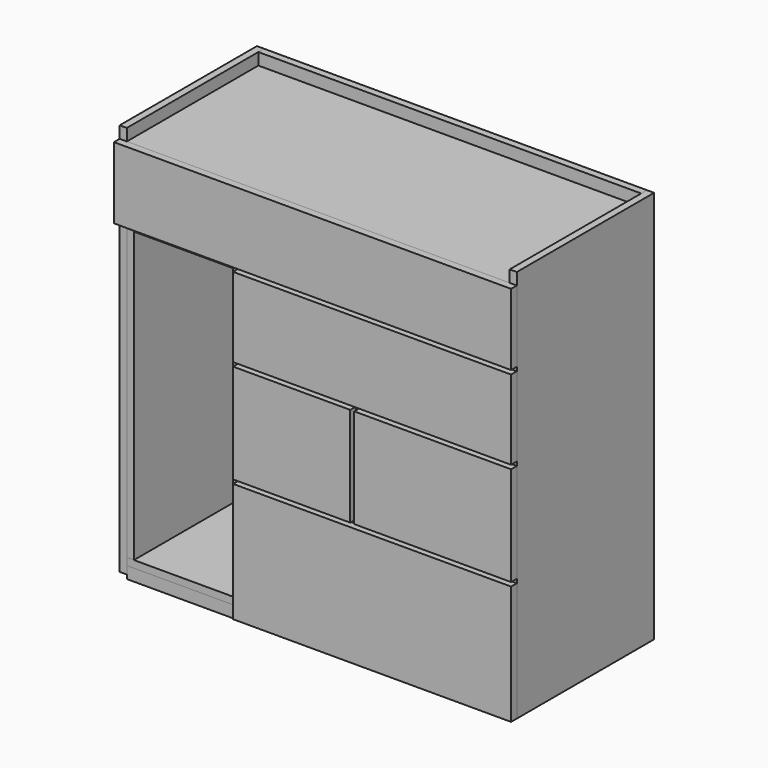
from build123d import *

# Parameters (mm, degrees)
F0_W          = 18
F0_H          = 414
F0_H_2        = 18
F1_DEPTH      = 990
F0_W_2        = 964
F2_DEPTH      = 990
F3_DEPTH      = 20
F3_DEPTH_BACK = 10
F4_W          = 982
F4_H          = 180
F4_W_2        = 18
F5_DEPTH      = 18
F4_W_3        = 700
F4_H_2        = 200
F4_W_4        = 395
F4_H_3        = 250
F4_H_4        = 300
F4_W_5        = 295
F6_W          = 964
F6_H          = 18
F7_DEPTH      = 414
F6_H_2        = 4
F6_W_2        = 18
F6_W_3        = 250
F6_H_3        = 192
F6_H_4        = 258
F6_H_5        = 242
F8_DEPTH      = 414
F9_R          = 10
F10_DEPTH     = 250
F11_W         = 250
F11_H         = 728
F12_DEPTH     = 12


# Not quite as in the source:
# - a feature names something its author has since deleted; it is built from what else it names


with BuildPart() as f1:
    # F0 (on Top) → F1 (new body)
    with BuildSketch(Plane.XY):
        with Locations((9, 207)):
            Rectangle(F0_W, F0_H)
        with Locations((9, 423)):
            Rectangle(F0_W, F0_H_2)
    extrude(amount=F1_DEPTH)


with BuildPart() as f1b:
    # F0 (on Top) → F1, piece 2 (new body)
    with BuildSketch(Plane.XY):
        with Locations((991, 423)):
            Rectangle(F0_W, F0_H_2)
        with Locations((991, 207)):
            Rectangle(F0_W, F0_H)
    extrude(amount=F1_DEPTH)


with BuildPart() as f2:
    # F0 (on Top) → F2 (new body, through all)
    with BuildSketch(Plane.XY):
        with Locations((500, 423)):
            Rectangle(F0_W_2, F0_H_2)
    extrude(amount=F2_DEPTH)


with BuildPart() as f3:
    # F0 (on Top) → F3 (new body, two sides)
    with BuildSketch(Plane.XY) as f3_sk:
        with Locations((500, 207)):
            Rectangle(F0_W_2, F0_H)
    extrude(amount=F3_DEPTH)
    extrude(f3_sk.sketch, amount=-F3_DEPTH_BACK)


with BuildPart() as f5:
    # F4 (on face) → F5 (new body)
    with BuildSketch(Plane.XZ):
        with Locations((509, 870)):
            Rectangle(F4_W, F4_H)
        with Locations((9, 870)):
            Rectangle(F4_W_2, F4_H)
    extrude(amount=F5_DEPTH)


with BuildPart() as f5b:
    # F4 (on face) → F5, piece 2 (new body)
    with BuildSketch(Plane.XZ):
        with Locations((650, 670)):
            Rectangle(F4_W_3, F4_H_2)
    extrude(amount=F5_DEPTH)


with BuildPart() as f5c:
    # F4 (on face) → F5, piece 3 (new body)
    with BuildSketch(Plane.XZ):
        with Locations((802.5, 435)):
            Rectangle(F4_W_4, F4_H_3)
    extrude(amount=F5_DEPTH)


with BuildPart() as f5d:
    # F4 (on face) → F5, piece 4 (new body)
    with BuildSketch(Plane.XZ):
        with Locations((650, 150)):
            Rectangle(F4_W_3, F4_H_4)
    extrude(amount=F5_DEPTH)


with BuildPart() as f5e:
    # F4 (on face) → F5, piece 5 (new body)
    with BuildSketch(Plane.XZ):
        with Locations((447.5, 435)):
            Rectangle(F4_W_5, F4_H_3)
    extrude(amount=F5_DEPTH)


with BuildPart() as f7:
    # F6 (on face) → F7 (new body, through all)
    with BuildSketch(Plane(origin=(0, 0, 0), x_dir=(-1, 0, 0), z_dir=(0, 1, 0))):
        with Locations((-500, 951)):
            Rectangle(F6_W, F6_H)
    extrude(amount=F7_DEPTH)


with BuildPart() as f7b:
    # F6 (on face) → F7, piece 2 (new body, through all)
    with BuildSketch(Plane(origin=(0, 0, 0), x_dir=(-1, 0, 0), z_dir=(0, 1, 0))):
        Polygon((-18, 780), (-982, 780), (-982, 766), (-304, 766), (-286, 766), (-36, 766), (-18, 766), align=None)
        with Locations((-500, 782)):
            Rectangle(F6_W, F6_H_2)
    extrude(amount=F7_DEPTH)


with BuildPart() as f7c:
    # F6 (on face) → F7, piece 3 (new body, through all)
    with BuildSketch(Plane(origin=(0, 0, 0), x_dir=(-1, 0, 0), z_dir=(0, 1, 0))):
        Polygon((-304, 556), (-304, 574), (-982, 574), (-982, 556), (-614, 556), (-596, 556), align=None)
    extrude(amount=F7_DEPTH)


with BuildPart() as f7d:
    # F6 (on face) → F7, piece 4 (new body, through all)
    with BuildSketch(Plane(origin=(0, 0, 0), x_dir=(-1, 0, 0), z_dir=(0, 1, 0))):
        Polygon((-304, 296), (-304, 314), (-596, 314), (-614, 314), (-982, 314), (-982, 296), align=None)
    extrude(amount=F7_DEPTH)


with BuildPart() as f7e:
    # F6 (on face) → F7, piece 5 (new body, through all)
    with BuildSketch(Plane(origin=(0, 0, 0), x_dir=(-1, 0, 0), z_dir=(0, 1, 0))):
        with Locations((-295, 29)):
            Rectangle(F6_W_2, F6_H)
        with Locations((-161, 29)):
            Rectangle(F6_W_3, F6_H)
        with Locations((-27, 29)):
            Rectangle(F6_W_2, F6_H)
    extrude(amount=F7_DEPTH)


with BuildPart() as f8:
    # F6 (on face) → F8 (new body, through all)
    with BuildSketch(Plane(origin=(0, 0, 0), x_dir=(-1, 0, 0), z_dir=(0, 1, 0))):
        with Locations((-295, 670)):
            Rectangle(F6_W_2, F6_H_3)
        with Locations((-295, 167)):
            Rectangle(F6_W_2, F6_H_4)
        with Locations((-295, 305)):
            Rectangle(F6_W_2, F6_H)
        with Locations((-295, 435)):
            Rectangle(F6_W_2, F6_H_5)
        with Locations((-295, 565)):
            Rectangle(F6_W_2, F6_H)
    extrude(amount=F8_DEPTH)


with BuildPart() as f8b:
    # F6 (on face) → F8, piece 2 (new body, through all)
    with BuildSketch(Plane(origin=(0, 0, 0), x_dir=(-1, 0, 0), z_dir=(0, 1, 0))):
        with Locations((-605, 435)):
            Rectangle(F6_W_2, F6_H_5)
    extrude(amount=F8_DEPTH)


with BuildPart() as f8c:
    # F6 (on face) → F8, piece 3 (new body, through all)
    with BuildSketch(Plane(origin=(0, 0, 0), x_dir=(-1, 0, 0), z_dir=(0, 1, 0))):
        with Locations((-27, 670)):
            Rectangle(F6_W_2, F6_H_3)
        with Locations((-27, 565)):
            Rectangle(F6_W_2, F6_H)
        with Locations((-27, 435)):
            Rectangle(F6_W_2, F6_H_5)
        with Locations((-27, 305)):
            Rectangle(F6_W_2, F6_H)
        with Locations((-27, 167)):
            Rectangle(F6_W_2, F6_H_4)
    extrude(amount=F8_DEPTH)


with BuildPart() as f10:
    # F9 (on face) → F10 (new body, through all)
    with BuildSketch(Plane.YZ.offset(36)):
        with Locations((207, 706)):
            Circle(F9_R)
    extrude(amount=F10_DEPTH)


with BuildPart() as f12:
    # F11 (on face) → F12 (new body)
    with BuildSketch(Plane.XZ.offset(-414)):
        with Locations((161, 402)):
            Rectangle(F11_W, F11_H)
    extrude(amount=F12_DEPTH)


solid = Compound([f1.part, f1b.part, f2.part, f3.part, f5.part, f5b.part, f5c.part, f5d.part, f5e.part, f7.part, f7b.part, f7c.part, f7d.part, f7e.part, f8.part, f8b.part, f8c.part, f10.part, f12.part])
